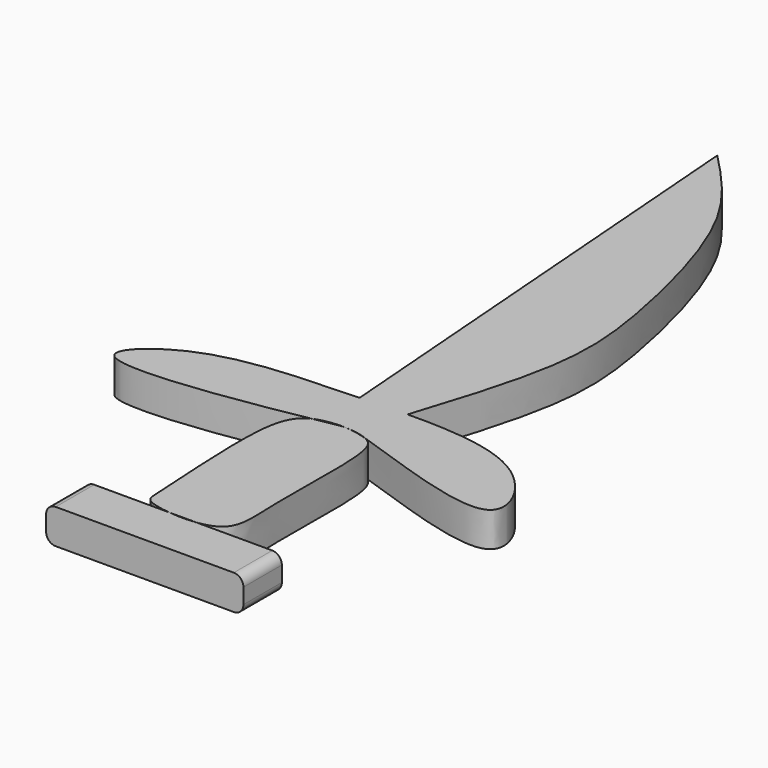
from build123d import *

# Parameters (mm, degrees)
F1_DEPTH = 4.572
F2_R     = 1.27
F3_R     = 1.27
F4_R     = 1.27
F5_R     = 1.27


with BuildPart() as f1:
    # F0 (on Top) → F1 (new body)
    with BuildSketch(Plane.XY):
        with BuildLine():
            add(Edge.make_bspline(
                [(-29.8993531615, -3.5077452194), (-31.6703462632, -4.3197464152), (-33.4416768807, -8.8355358115), (-31.9008991214, -26.0699501287), (-32.073712776, -27.9811963987), (-31.2356371433, -28.3960327506)],
                knots=[0.6307578864, 0.6307578864, 0.6307578864, 0.6307578864, 0.7429048342, 0.9308873949, 1, 1, 1, 1], degree=3))
            add(Edge.make_bspline(
                [(-31.2356371433, -28.3960327506), (-30.6428751172, -28.6894421123), (-29.6076188044, -28.9333524282), (-28.4280432172, -29.0641747415)],
                knots=[0, 0, 0, 0, 0.0488826142, 0.0488826142, 0.0488826142, 0.0488826142], degree=3))
            Line((-28.4280432172, -29.0641747415), (-24.8331572694, -29.0641747415))
            add(Edge.make_bspline(
                [(-24.8331572694, -29.0641747415), (-23.9456810218, -28.9502333326), (-20.4658515137, -28.0253654937), (-21.4945827069, -21.0427899664), (-20.5497100233, -6.2066091766), (-22.0747955225, -3.9219376818), (-22.9658381019, -3.5077452194)],
                knots=[0.0966734598, 0.0966734598, 0.0966734598, 0.0966734598, 0.1335391331, 0.2562819752, 0.4339266036, 0.5047742263, 0.5047742263, 0.5047742263, 0.5047742263], degree=3))
            add(Edge.make_bspline(
                [(-29.8993531615, -3.5077452194), (-26.5539886397, -2.8472558093), (-25.9297526703, -2.6050307792), (-22.9658381019, -3.5077452194)],
                knots=[0.4512013353, 0.4512013353, 0.4512013353, 0.4512013353, 0.548270897, 0.548270897, 0.548270897, 0.548270897], degree=3))
        make_face()
    extrude(amount=F1_DEPTH)


with BuildPart() as f1b:
    # F0 (on Top) → F1, piece 2 (new body)
    with BuildSketch(Plane.XY):
        with BuildLine():
            add(Edge.make_bspline(
                [(-28.4280432172, -29.0641747415), (-27.2748128564, -29.1920752043), (-25.9836378271, -29.2118827799), (-24.8331572694, -29.0641747415)],
                knots=[0.0488826142, 0.0488826142, 0.0488826142, 0.0488826142, 0.0966734598, 0.0966734598, 0.0966734598, 0.0966734598], degree=3))
            Line((-28.4280432172, -29.0641747415), (-39.5874110982, -29.0641747415))
            Line((-39.5874110982, -29.0641747415), (-39.5874110982, -35.4115255177))
            Line((-39.5874110982, -35.4115255177), (-13.5298753157, -35.4115255177))
            Line((-13.5298753157, -35.4115255177), (-13.5298753157, -29.0641747415))
            Line((-13.5298753157, -29.0641747415), (-24.8331572694, -29.0641747415))
        make_face()
    extrude(amount=F1_DEPTH)

    # F2
    f2_edges = [f1b.edges().sort_by_distance(p)[0] for p in [
        (-39.587411, -32.23785, 4.572),
    ]]
    fillet(f2_edges, radius=F2_R)

    # F3
    f3_edges = [f1b.edges().sort_by_distance(p)[0] for p in [
        (-39.587411, -32.23785, 0),
    ]]
    fillet(f3_edges, radius=F3_R)

    # F4
    f4_edges = [f1b.edges().sort_by_distance(p)[0] for p in [
        (-13.529875, -32.23785, 0),
    ]]
    fillet(f4_edges, radius=F4_R)

    # F5
    f5_edges = [f1b.edges().sort_by_distance(p)[0] for p in [
        (-13.529875, -32.23785, 4.572),
    ]]
    fillet(f5_edges, radius=F5_R)


with BuildPart() as f1c:
    # F0 (on Top) → F1, piece 3 (new body)
    with BuildSketch(Plane.XY):
        with BuildLine():
            add(Edge.make_bspline(
                [(-29.0641766042, 3.1736744568), (-36.9995706334, 2.8839279058), (-48.5838670621, 2.7774177029), (-60.872789795, -8.9698768638), (-36.2249289881, -4.7566303017), (-29.8993531615, -3.5077452194)],
                knots=[0, 0, 0, 0, 0.1694125769, 0.2676575484, 0.4512013353, 0.4512013353, 0.4512013353, 0.4512013353], degree=3))
            add(Edge.make_bspline(
                [(-22.9658381019, -3.5077452194), (-23.0955860892, -3.4474331315), (-24.7982012469, -2.7723188561), (-28.0727680061, -2.67025504), (-29.8993531615, -3.5077452194)],
                knots=[0.5047742263, 0.5047742263, 0.5047742263, 0.5047742263, 0.5150906092, 0.6307578864, 0.6307578864, 0.6307578864, 0.6307578864], degree=3))
            add(Edge.make_bspline(
                [(-22.9658381019, -3.5077452194), (-17.8740876083, -5.0585310435), (1.968128388, -13.2122424462), (-5.6130342206, 2.6563547922), (-16.6332168416, 3.4628720663), (-22.8846012587, 3.3684871276)],
                knots=[0.548270897, 0.548270897, 0.548270897, 0.548270897, 0.7150280613, 0.824083244, 0.9564302387, 0.9564302387, 0.9564302387, 0.9564302387], degree=3))
            add(Edge.make_bspline(
                [(-22.8846012587, 3.3684871276), (-24.942610411, 3.3374147995), (-27.023340973, 3.2481918762), (-29.0641766042, 3.1736744568)],
                knots=[0.9564302387, 0.9564302387, 0.9564302387, 0.9564302387, 1, 1, 1, 1], degree=3))
        make_face()
        with BuildLine():
            Line((-34.0752415359, 68.4845522046), (-29.0641766042, 3.1736744568))
            add(Edge.make_bspline(
                [(-22.8846012587, 3.3684871276), (-24.942610411, 3.3374147995), (-27.023340973, 3.2481918762), (-29.0641766042, 3.1736744568)],
                knots=[0.9564302387, 0.9564302387, 0.9564302387, 0.9564302387, 1, 1, 1, 1], degree=3))
            add(Edge.make_bspline(
                [(-22.8846012587, 3.3684871276), (-20.7332880928, 10.0991858385), (-16.7589477096, 22.5245770204), (-18.2384375016, 36.5615536627), (-23.7070572199, 57.7855641977), (-30.8381753552, 65.1442313261), (-34.0752415359, 68.4845522046)],
                knots=[0, 0, 0, 0, 0.2673865788, 0.4938609679, 0.7702621718, 1, 1, 1, 1], degree=3))
        make_face()
    extrude(amount=F1_DEPTH)


solid = Compound([f1.part, f1b.part, f1c.part])
